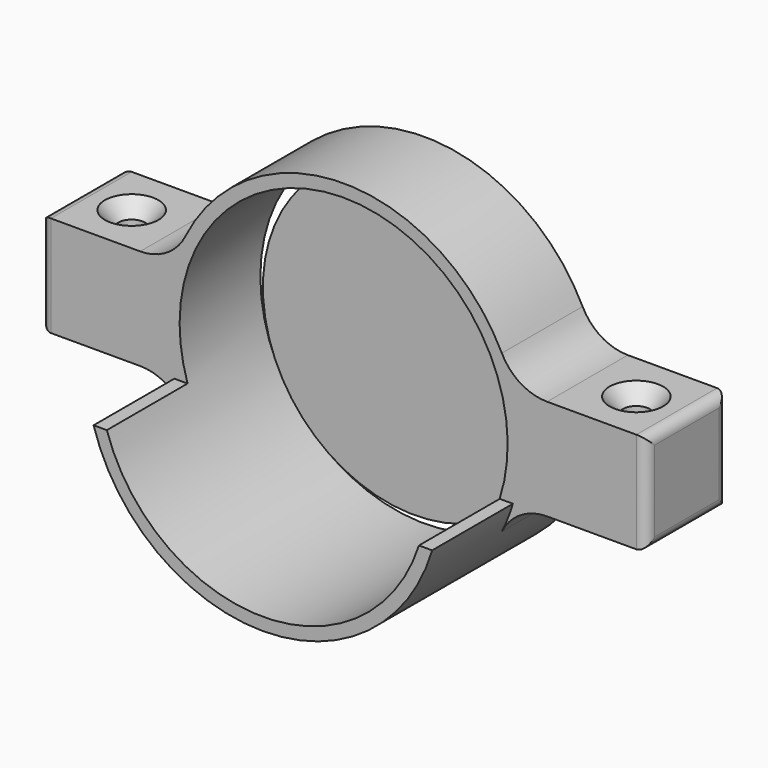
from build123d import *

# Parameters (mm, degrees)
F1_DEPTH       = 50.8
F2_DEPTH       = 25.4
F4_D           = 6.7564
F4_CSINK_D     = 13.4874
F4_CSINK_ANGLE = 82
F5_R           = 12.7
F6_R           = 2.54
F7_R           = 41.275
F8_DEPTH       = 72.39
F9_R           = 38.1
F10_DEPTH      = 3.175


with BuildPart() as f1:
    # F0 (on Front) → F1 (new body)
    with BuildSketch(Plane.XZ):
        with BuildLine():
            ThreePointArc((-42.5970949714, -12.7), (0, -44.45), (42.5970949714, -12.7))
            Line((42.5970949714, -12.7), (-42.5970949714, -12.7))
        make_face()
    extrude(amount=F1_DEPTH)

    # F0 (on Front) → F2 (join)
    with BuildSketch(Plane.XZ):
        with BuildLine():
            ThreePointArc((42.5970949714, -12.7), (43.9843345492, -6.4172279265), (44.45, 0))
            ThreePointArc((44.45, 0), (43.9843345492, 6.4172279265), (42.5970949714, 12.7))
            Line((42.5970949714, 12.7), (-42.5970949714, 12.7))
            ThreePointArc((-42.5970949714, 12.7), (-44.45, 0), (-42.5970949714, -12.7))
            Line((-42.5970949714, -12.7), (42.5970949714, -12.7))
        make_face()
        with BuildLine():
            ThreePointArc((42.5970949714, 12.7), (43.9843345492, 6.4172279265), (44.45, 0))
            ThreePointArc((44.45, 0), (43.9843345492, -6.4172279265), (42.5970949714, -12.7))
            Line((42.5970949714, -12.7), (76.2, -12.7))
            Line((76.2, -12.7), (76.2, 12.7))
            Line((76.2, 12.7), (42.5970949714, 12.7))
        make_face()
        with BuildLine():
            Line((-42.5970949714, 12.7), (42.5970949714, 12.7))
            ThreePointArc((42.5970949714, 12.7), (0, 44.45), (-42.5970949714, 12.7))
        make_face()
        with BuildLine():
            ThreePointArc((-42.5970949714, -12.7), (0, -44.45), (42.5970949714, -12.7))
            Line((42.5970949714, -12.7), (-42.5970949714, -12.7))
        make_face()
        with BuildLine():
            ThreePointArc((-42.5970949714, -12.7), (-44.45, 0), (-42.5970949714, 12.7))
            Line((-42.5970949714, 12.7), (-76.2, 12.7))
            Line((-76.2, 12.7), (-76.2, -12.7))
            Line((-76.2, -12.7), (-42.5970949714, -12.7))
        make_face()
    extrude(amount=F2_DEPTH)

    # F4 (through all)
    with Locations(Plane.XY.offset(12.7)):
        with Locations((-63.5, -12.7), (63.5, -12.7)):
            CounterSinkHole(F4_D / 2, F4_CSINK_D / 2, counter_sink_angle=F4_CSINK_ANGLE)

    # F5
    f5_edges = [f1.edges().sort_by_distance(p)[0] for p in [
        (-42.597095, -12.7, -12.7),
        (42.597095, -12.7, -12.7),
        (-42.597095, -12.7, 12.7),
        (42.597095, -12.7, 12.7),
    ]]
    fillet(f5_edges, radius=F5_R)

    # F6
    f6_edges = [f1.edges().sort_by_distance(p)[0] for p in [
        (-76.2, -25.4, 0),
        (-76.2, -12.7, 12.7),
        (-76.2, -12.7, -12.7),
        (-76.2, 0, 0),
        (76.2, -12.7, 12.7),
        (76.2, -12.7, -12.7),
        (76.2, 0, 0),
        (76.2, -25.4, 0),
    ]]
    fillet(f6_edges, radius=F6_R)

    # F7 (on face) → F8 (cut, symmetric)
    with BuildSketch(Plane(origin=(0, 0, 0), x_dir=(-1, 0, 0), z_dir=(0, 1, 0))):
        Circle(F7_R)
    extrude(amount=F8_DEPTH, both=True, mode=Mode.SUBTRACT)


with BuildPart() as f10:
    # F9 (on Front) → F10 (new body)
    with BuildSketch(Plane.XZ):
        Circle(F9_R)
    extrude(amount=F10_DEPTH)


solid = Compound([f1.part, f10.part])
